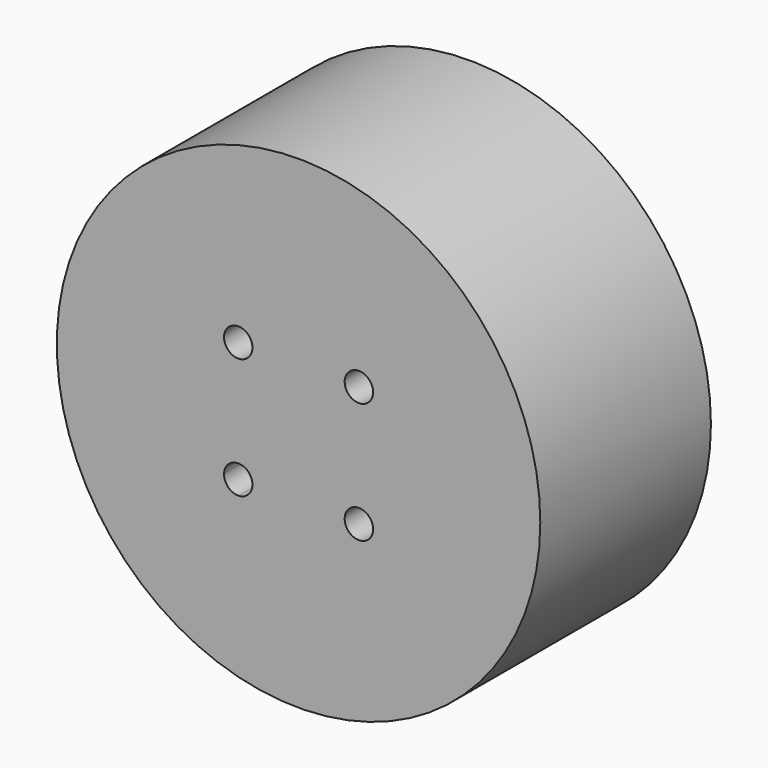
from build123d import *

# Parameters (mm, degrees)
F0_R     = 17
F0_R_2   = 1.5
F0_R_3   = 1
F1_DEPTH = 15
F2_START = 10
F2_DEPTH = 15
F3_DEPTH = 5


# Not quite as in the source:
# - a feature names something its author has since deleted; it is built from what else it names


with BuildPart() as f1:
    # F0 (on Front) → F1 (new body)
    with BuildSketch(Plane.XZ):
        Circle(F0_R)
        with BuildLine():
            ThreePointArc((-4.2152867015, -5.2422664968), (-4.1715341961, -5.447511614), (-4.1568542495, -5.6568542495))
            ThreePointArc((-4.1568542495, -5.6568542495), (-6.8551617286, -6.5591065343), (-5.2422664968, -4.2152867015))
            ThreePointArc((-5.2422664968, -4.2152867015), (-4.2289624147, -3.2427342391), (-3.2426406871, -4.2426406871))
            ThreePointArc((-3.2426406871, -4.2426406871), (-3.525928058, -4.9400093179), (-4.2152867015, -5.2422664968))
        make_face(mode=Mode.SUBTRACT)
        with Locations((6.7175144213, -6.7175144213)):
            Circle(F0_R_2, mode=Mode.SUBTRACT)
        with Locations((4.2426406871, -4.2426406871)):
            Circle(F0_R_3, mode=Mode.SUBTRACT)
        with Locations((-4.2426406871, 4.2426406871)):
            Circle(F0_R_3, mode=Mode.SUBTRACT)
        with Locations((-6.7175144213, 6.7175144213)):
            Circle(F0_R_2, mode=Mode.SUBTRACT)
        with BuildLine():
            ThreePointArc((4.2152867015, 5.2422664968), (5.447511614, 7.1421743029), (7.1568542495, 5.6568542495))
            ThreePointArc((7.1568542495, 5.6568542495), (6.5591065343, 4.4585467704), (5.2422664968, 4.2152867015))
            ThreePointArc((5.2422664968, 4.2152867015), (3.5355339059, 3.5355339059), (4.2152867015, 5.2422664968))
        make_face(mode=Mode.SUBTRACT)
        with BuildLine():
            ThreePointArc((5.2422664968, 4.2152867015), (6.5591065343, 4.4585467704), (7.1568542495, 5.6568542495))
            ThreePointArc((7.1568542495, 5.6568542495), (5.447511614, 7.1421743029), (4.2152867015, 5.2422664968))
            ThreePointArc((4.2152867015, 5.2422664968), (4.9400093179, 4.9593533163), (5.2426406871, 4.2426406871))
            ThreePointArc((5.2426406871, 4.2426406871), (5.2425471352, 4.2289624147), (5.2422664968, 4.2152867015))
        make_face()
        with BuildLine():
            ThreePointArc((5.2422664968, 4.2152867015), (4.5961940777, 4.5961940777), (4.2152867015, 5.2422664968))
            ThreePointArc((4.2152867015, 5.2422664968), (3.5355339059, 3.5355339059), (5.2422664968, 4.2152867015))
        make_face()
        with BuildLine():
            ThreePointArc((-5.2422664968, -4.2152867015), (-6.8551617286, -6.5591065343), (-4.1568542495, -5.6568542495))
            ThreePointArc((-4.1568542495, -5.6568542495), (-4.1715341961, -5.447511614), (-4.2152867015, -5.2422664968))
            ThreePointArc((-4.2152867015, -5.2422664968), (-4.9497474683, -4.9497474683), (-5.2422664968, -4.2152867015))
        make_face()
        with BuildLine():
            ThreePointArc((-5.2422664968, -4.2152867015), (-4.9497474683, -4.9497474683), (-4.2152867015, -5.2422664968))
            ThreePointArc((-4.2152867015, -5.2422664968), (-4.5961940777, -4.5961940777), (-5.2422664968, -4.2152867015))
        make_face()
        with BuildLine():
            ThreePointArc((-5.2422664968, -4.2152867015), (-4.5961940777, -4.5961940777), (-4.2152867015, -5.2422664968))
            ThreePointArc((-4.2152867015, -5.2422664968), (-3.525928058, -4.9400093179), (-3.2426406871, -4.2426406871))
            ThreePointArc((-3.2426406871, -4.2426406871), (-4.2289624147, -3.2427342391), (-5.2422664968, -4.2152867015))
        make_face()
        with BuildLine():
            ThreePointArc((5.2426406871, 4.2426406871), (4.9400093179, 4.9593533163), (4.2152867015, 5.2422664968))
            ThreePointArc((4.2152867015, 5.2422664968), (4.5961940777, 4.5961940777), (5.2422664968, 4.2152867015))
            ThreePointArc((5.2422664968, 4.2152867015), (5.2425471352, 4.2289624147), (5.2426406871, 4.2426406871))
        make_face()
        with Locations((4.2426406871, -4.2426406871)):
            Circle(F0_R_3)
        with Locations((-4.2426406871, 4.2426406871)):
            Circle(F0_R_3)
        with Locations((-6.7175144213, 6.7175144213)):
            Circle(F0_R_2)
        with Locations((6.7175144213, -6.7175144213)):
            Circle(F0_R_2)
    extrude(amount=F1_DEPTH)

    # F0 (on Front) → F2 (cut)
    with BuildSketch(Plane.XZ.offset(F2_START)):
        with BuildLine():
            ThreePointArc((-5.2422664968, -4.2152867015), (-4.5961940777, -4.5961940777), (-4.2152867015, -5.2422664968))
            ThreePointArc((-4.2152867015, -5.2422664968), (-3.525928058, -4.9400093179), (-3.2426406871, -4.2426406871))
            ThreePointArc((-3.2426406871, -4.2426406871), (-4.2289624147, -3.2427342391), (-5.2422664968, -4.2152867015))
        make_face()
        with BuildLine():
            ThreePointArc((-5.2422664968, -4.2152867015), (-4.9497474683, -4.9497474683), (-4.2152867015, -5.2422664968))
            ThreePointArc((-4.2152867015, -5.2422664968), (-4.5961940777, -4.5961940777), (-5.2422664968, -4.2152867015))
        make_face()
        with Locations((4.2426406871, -4.2426406871)):
            Circle(F0_R_3)
        with BuildLine():
            ThreePointArc((5.2422664968, 4.2152867015), (4.5961940777, 4.5961940777), (4.2152867015, 5.2422664968))
            ThreePointArc((4.2152867015, 5.2422664968), (3.5355339059, 3.5355339059), (5.2422664968, 4.2152867015))
        make_face()
        with BuildLine():
            ThreePointArc((5.2426406871, 4.2426406871), (4.9400093179, 4.9593533163), (4.2152867015, 5.2422664968))
            ThreePointArc((4.2152867015, 5.2422664968), (4.5961940777, 4.5961940777), (5.2422664968, 4.2152867015))
            ThreePointArc((5.2422664968, 4.2152867015), (5.2425471352, 4.2289624147), (5.2426406871, 4.2426406871))
        make_face()
        with Locations((-4.2426406871, 4.2426406871)):
            Circle(F0_R_3)
    extrude(amount=F2_DEPTH, mode=Mode.SUBTRACT)

    # F0 (on Front) → F3 (cut)
    with BuildSketch(Plane.XZ):
        with BuildLine():
            ThreePointArc((5.2422664968, 4.2152867015), (6.5591065343, 4.4585467704), (7.1568542495, 5.6568542495))
            ThreePointArc((7.1568542495, 5.6568542495), (5.447511614, 7.1421743029), (4.2152867015, 5.2422664968))
            ThreePointArc((4.2152867015, 5.2422664968), (4.9400093179, 4.9593533163), (5.2426406871, 4.2426406871))
            ThreePointArc((5.2426406871, 4.2426406871), (5.2425471352, 4.2289624147), (5.2422664968, 4.2152867015))
        make_face()
        with BuildLine():
            ThreePointArc((5.2426406871, 4.2426406871), (4.9400093179, 4.9593533163), (4.2152867015, 5.2422664968))
            ThreePointArc((4.2152867015, 5.2422664968), (4.5961940777, 4.5961940777), (5.2422664968, 4.2152867015))
            ThreePointArc((5.2422664968, 4.2152867015), (5.2425471352, 4.2289624147), (5.2426406871, 4.2426406871))
        make_face()
        with BuildLine():
            ThreePointArc((-5.2422664968, -4.2152867015), (-6.8551617286, -6.5591065343), (-4.1568542495, -5.6568542495))
            ThreePointArc((-4.1568542495, -5.6568542495), (-4.1715341961, -5.447511614), (-4.2152867015, -5.2422664968))
            ThreePointArc((-4.2152867015, -5.2422664968), (-4.9497474683, -4.9497474683), (-5.2422664968, -4.2152867015))
        make_face()
        with BuildLine():
            ThreePointArc((-5.2422664968, -4.2152867015), (-4.9497474683, -4.9497474683), (-4.2152867015, -5.2422664968))
            ThreePointArc((-4.2152867015, -5.2422664968), (-4.5961940777, -4.5961940777), (-5.2422664968, -4.2152867015))
        make_face()
        with Locations((6.7175144213, -6.7175144213)):
            Circle(F0_R_2)
        with Locations((-6.7175144213, 6.7175144213)):
            Circle(F0_R_2)
    extrude(amount=F3_DEPTH, mode=Mode.SUBTRACT)


solid = f1.part
